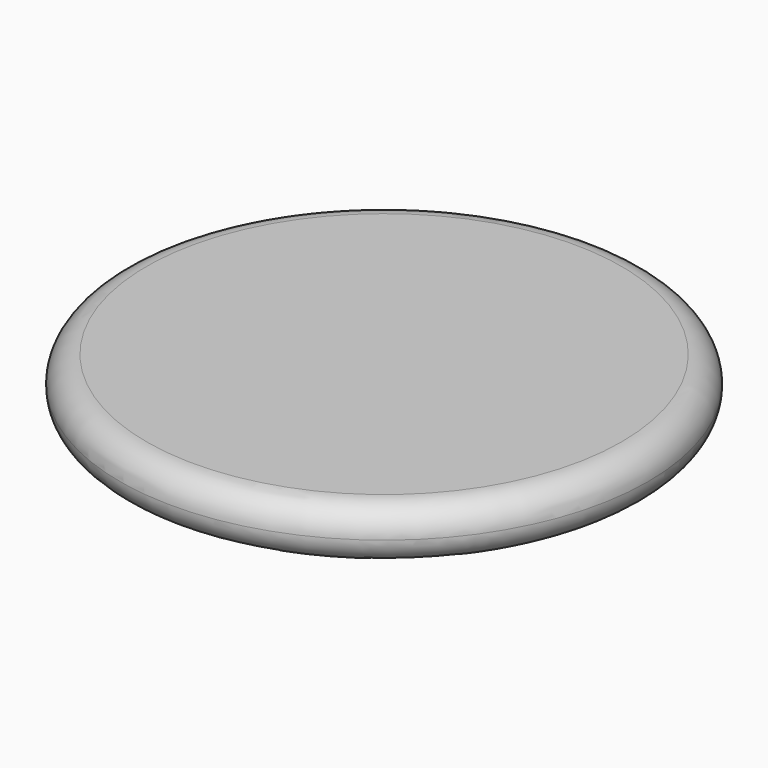
from build123d import *

# Parameters (mm, degrees)
F0_R     = 50
F1_DEPTH = 10
F2_R     = 4.99999
F3_W     = 9.3445703387
F3_H     = 114.5939677954
F3_W_2   = 10.3282090276
F3_H_2   = 115.5776083469
F3_W_3   = 9.3445708044
F3_H_3   = 117.5448857248
F3_H_4   = 117.0530617237
F4_DEPTH = 1


# Not quite as in the source:
# - a fillet or chamfer is up to 0.001 mm smaller than in the source, because OpenCascade refuses the exact size


with BuildPart() as f1:
    # F0 (on Top) → F1 (new body)
    with BuildSketch(Plane.XY):
        Circle(F0_R)
    extrude(amount=F1_DEPTH)

    # F2 (radius 5 in the source; OpenCascade refuses exactly that, so slightly less here)
    f2_edges = [f1.edges().sort_by_distance(p)[0] for p in [
        (-50, 0, 0),
        (-50, 0, 10),
    ]]
    fillet(f2_edges, radius=F2_R)

    # F3 (on face) → F4 (cut)
    with BuildSketch(Plane(origin=(0, 0, 0), x_dir=(1, 0, 0), z_dir=(0, 0, -1))):
        with Locations((-36.148738116, -1.2295395136)):
            Rectangle(F3_W, F3_H)
        with Locations((-12.5413937494, -1.7213597894)):
            Rectangle(F3_W_2, F3_H_2)
        with Locations((11.5577613469, -2.2131819278)):
            Rectangle(F3_W_3, F3_H_3)
        with Locations((32.7060082927, -2.9509104788)):
            Rectangle(F3_W_2, F3_H_4)
    extrude(amount=-F4_DEPTH, mode=Mode.SUBTRACT)


solid = f1.part
